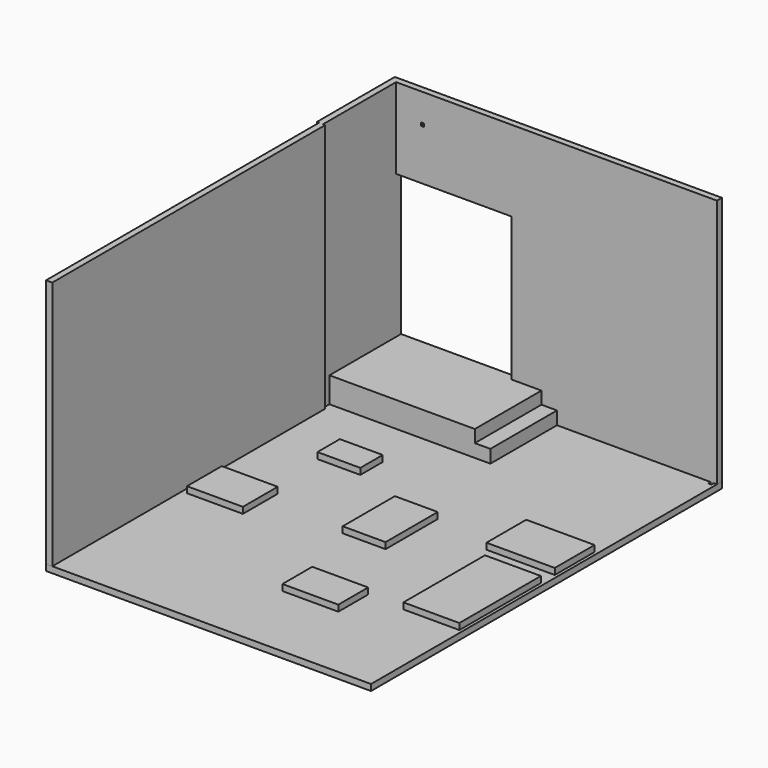
from build123d import *

# Parameters (mm, degrees)
F0_W      = 5490
F0_H      = 4020
F1_DEPTH  = 100
F3_W      = 1470
F3_H      = 4020
F4_DEPTH  = 100
F6_W      = 1855
F6_H      = 2720
F7_DEPTH  = 100
F8_W      = 1855
F8_H      = 2720
F9_DEPTH  = 100
F12_DEPTH = 100
F13_W     = 1100
F13_H     = 800
F13_W_2   = 900
F13_H_2   = 1640
F13_H_3   = 600
F13_W_3   = 690
F13_H_4   = 1050
F13_H_5   = 700
F13_H_6   = 450
F14_DEPTH = 100
F15_W     = 2590
F15_H     = 1340
F16_DEPTH = 210
F17_W     = 2340
F17_H     = 1340
F18_DEPTH = 200
F19_W     = 1855
F19_H     = 100
F20_DEPTH = 510
F23_W     = 50
F23_H     = 50
F24_DEPTH = 100
F25_W     = 50
F25_H     = 50
F26_DEPTH = 100


with BuildPart() as f1:
    # F0 (on Right) → F1 (new body)
    with BuildSketch(Plane.YZ):
        Rectangle(F0_W, F0_H)
    extrude(amount=-F1_DEPTH)

    # F3 (on offset) → F4 (join)
    with BuildSketch(Plane.YZ.offset(-35)):
        with Locations((3480, 0)):
            Rectangle(F3_W, F3_H)
    extrude(amount=-F4_DEPTH)

    # F6 (on offset) → F7 (join)
    with BuildSketch(Plane.XZ.offset(-4215)):
        Polygon((5130, 2010), (-35, 2010), (-35, 710), (1820, 710), (1820, -2010), (5130, -2010), align=None)
        Polygon((-35, 710), (-35, 2010), (-135, 2010), (-135, -2010), (-35, -2010), align=None)
        with Locations((892.5, -650)):
            Rectangle(F6_W, F6_H)
    extrude(amount=-F7_DEPTH)

    # F8 (on face) → F9 (cut)
    with BuildSketch(Plane.XZ.offset(-4215)):
        with Locations((892.5, -650)):
            Rectangle(F8_W, F8_H)
    extrude(amount=-F9_DEPTH, mode=Mode.SUBTRACT)

    # F25 (on face) → F26 (cut)
    with BuildSketch(Plane.XZ.offset(-4215)):
        with Locations((390, 1545)):
            Rectangle(F25_W, F25_H)
    extrude(amount=-F26_DEPTH, mode=Mode.SUBTRACT)


with BuildPart() as f12:
    # F11 (on offset) → F12 (new body)
    with BuildSketch(Plane.XY.offset(-2010)):
        Polygon((-100, 2745), (-100, -2745), (0, -2745), (5130, -2745), (5130, 4215), (5130, 4315), (1820, 4315), (-35, 4315), (-135, 4315), (-135, 2745), align=None)
    extrude(amount=-F12_DEPTH)

    # F13 (on face) → F14 (join)
    with BuildSketch(Plane.XY.offset(-2010)):
        with Locations((4530, 1415)):
            Rectangle(F13_W, F13_H)
        with Locations((4630, -85)):
            Rectangle(F13_W_2, F13_H_2)
        with Locations((3130, -1165)):
            Rectangle(F13_W_2, F13_H_3)
        with Locations((2635, 760)):
            Rectangle(F13_W_3, F13_H_4)
        with Locations((530, 215)):
            Rectangle(F13_W_2, F13_H_5)
        with Locations((1125, 1840)):
            Rectangle(F13_W_3, F13_H_6)
    extrude(amount=F14_DEPTH)

    # F15 (on face) → F16 (join)
    with BuildSketch(Plane.XY.offset(-2010)):
        with Locations((1260, 3545)):
            Rectangle(F15_W, F15_H)
    extrude(amount=F16_DEPTH)

    # F17 (on face) → F18 (join)
    with BuildSketch(Plane.XY.offset(-1800)):
        with Locations((1135, 3545)):
            Rectangle(F17_W, F17_H)
    extrude(amount=F18_DEPTH)

    # F19 (on face) → F20 (join)
    with BuildSketch(Plane.XY.offset(-1600)):
        with Locations((892.5, 4265)):
            Rectangle(F19_W, F19_H)
    extrude(amount=-F20_DEPTH)

    # F21: union 

    # F23 (on face) → F24 (cut)
    with BuildSketch(Plane.XY.offset(-2010)):
        with Locations((5055, 4190)):
            Rectangle(F23_W, F23_H)
    extrude(amount=-F24_DEPTH, mode=Mode.SUBTRACT)


solid = Compound([f1.part, f12.part])
